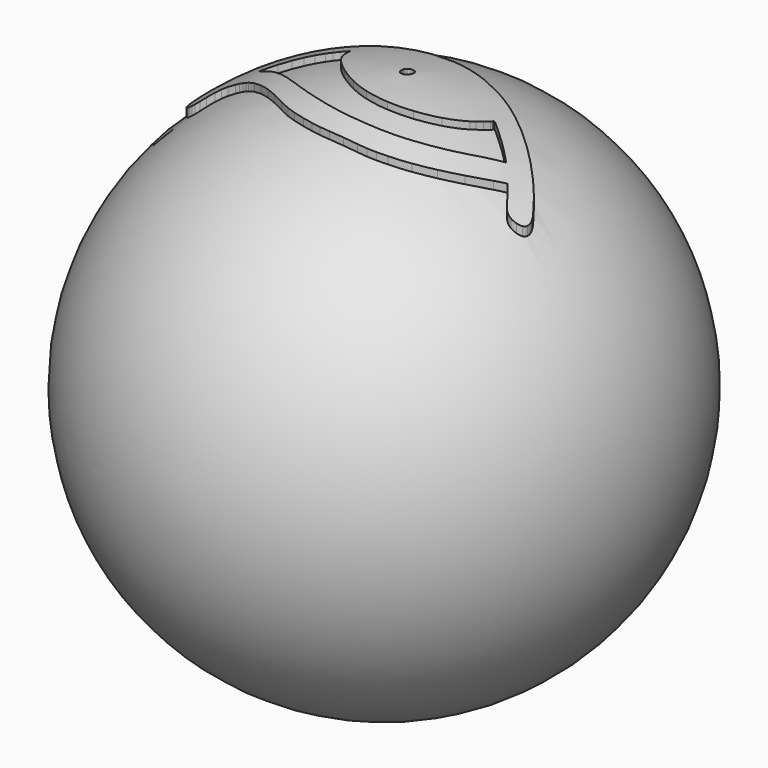
from build123d import *

# Parameters (mm, degrees)
F2_SCALE  = 33.3
F4_DEPTH  = 350
F5_SCALE  = 0.03
F8_SCALE  = 1.4
F9_R      = 2
F10_DEPTH = 25


# Not quite as in the source:
# - ends of sketch curves that miss each other by under 0.0002 mm in the source are joined


with BuildPart() as f1:
    # F0 (on Top) → F1 (revolve)
    with BuildSketch(Plane.XY):
        with BuildLine():
            ThreePointArc((0, 10), (-10, 0), (0, -10))
            Line((0, -10), (0, 10))
        make_face()
    revolve(axis=Axis((0, 0, 0), (0, 1, 0)))


with BuildPart() as f1_1:
    # F2: moved
    add(f1.part.scale(F2_SCALE))

    # F3 (on Top) → F4 (join)
    with BuildSketch(Plane.XY):
        with BuildLine():
            ThreePointArc((10.0534840034, 96.9614781182), (-2.8301346595, 96.9747207616), (-15.6947390095, 96.2748921162))
            ThreePointArc((-15.6947390095, 96.2748921162), (-24.8751298312, 95.2803343458), (-33.991766952, 93.8121217445))
            ThreePointArc((-33.991766952, 93.8121217445), (-43.5504868945, 91.8004399256), (-53.0120990138, 89.3727070494))
            ThreePointArc((-53.0120990138, 89.3727070494), (-62.3941886789, 86.5234517907), (-71.6431770265, 83.2679830704))
            ThreePointArc((-71.6431770265, 83.2679830704), (-80.3024909146, 79.7548321438), (-88.7739972032, 75.8102754091))
            ThreePointArc((-88.7739972032, 75.8102754091), (-102.8123104581, 68.2085488829), (-116.2787087414, 59.6343666239))
            ThreePointArc((-116.2787087414, 59.6343666239), (-129.8649070153, 49.6780948633), (-142.827490195, 38.9224652211))
            ThreePointArc((-142.827490195, 38.9224652211), (-156.8673095819, 25.8818104455), (-170.2157531103, 12.1342921017))
            ThreePointArc((-170.2157531103, 12.1342921017), (-185.5506121287, -5.0061794181), (-200.3640161811, -22.5992668521))
            ThreePointArc((-200.3640161811, -22.5992668521), (-204.2556653518, -27.3979139103), (-208.1144591023, -32.2230209187))
            ThreePointArc((-208.1144591023, -32.2230209187), (-209.6806871871, -34.3340096505), (-211.1049830246, -36.5432459852))
            ThreePointArc((-211.1049830246, -36.5432459852), (-211.8903487056, -38.1080067712), (-212.4343023025, -39.7721551716))
            ThreePointArc((-212.4343023025, -39.7721551716), (-212.7727330789, -41.6217988462), (-212.886093, -43.498729))
            ThreePointArc((-212.886093, -43.498729), (-212.7053479315, -45.3625594436), (-212.1698450767, -47.1569310312))
            ThreePointArc((-212.1698450767, -47.1569310312), (-211.2496275997, -49.0288969817), (-210.0765223808, -50.7536813001))
            ThreePointArc((-210.0765223808, -50.7536813001), (-208.6303513581, -52.3522530467), (-206.981032979, -53.7402699713))
            ThreePointArc((-206.981032979, -53.7402699713), (-205.2320729108, -54.8208646921), (-203.3361079867, -55.6157629597))
            ThreePointArc((-203.3361079867, -55.6157629597), (-201.3422328116, -56.0863212361), (-199.2969970047, -56.2045318412))
            ThreePointArc((-199.2969970047, -56.2045318412), (-197.4275801661, -55.9408822607), (-195.6618639687, -55.2726930612))
            ThreePointArc((-195.6618639687, -55.2726930612), (-193.6718494664, -54.0492698967), (-191.8979606388, -52.52932236))
            ThreePointArc((-191.8979606388, -52.52932236), (-189.5399689495, -50.0368818855), (-187.3149011588, -47.4250898717))
            ThreePointArc((-187.3149011588, -47.4250898717), (-184.5776350656, -44.2864403575), (-181.612206547, -41.3624054954))
            ThreePointArc((-181.612206547, -41.3624054954), (-179.0131248493, -39.3175211967), (-176.1404878573, -37.6790052998))
            ThreePointArc((-176.1404878573, -37.6790052998), (-172.9686200832, -36.4355960849), (-169.65328502, -35.6511438773))
            ThreePointArc((-169.65328502, -35.6511438773), (-165.1982751687, -35.067458336), (-160.7153950073, -34.7648247958))
            ThreePointArc((-160.7153950073, -34.7648247958), (-158.1528140465, -34.7037638823), (-155.5895059941, -34.7049725349))
            ThreePointArc((-155.5895059941, -34.7049725349), (-153.4579068829, -34.7765835211), (-151.3311820401, -34.9374694148))
            ThreePointArc((-151.3311820401, -34.9374694148), (-149.2878923738, -35.180741935), (-147.2573030885, -35.5137904739))
            ThreePointArc((-147.2573030885, -35.5137904739), (-144.9787497299, -35.975458744), (-142.7153951261, -36.5066545025))
            ThreePointArc((-142.7153951261, -36.5066545025), (-137.7060507754, -37.9788293633), (-132.8304160593, -39.8467201381))
            ThreePointArc((-132.8304160593, -39.8467201381), (-126.177935546, -42.8259254875), (-119.6189671008, -46.0057202002))
            ThreePointArc((-119.6189671008, -46.0057202002), (-111.9353070881, -50.0083471014), (-104.3637867666, -54.2192535934))
            ThreePointArc((-104.3637867666, -54.2192535934), (-96.07539311, -59.0890561452), (-87.8860931987, -64.1237173161))
            ThreePointArc((-87.8860931987, -64.1237173161), (-78.6401870334, -69.8346933419), (-69.3050959968, -75.3986939946))
            ThreePointArc((-69.3050959968, -75.3986939946), (-62.777455601, -79.0174912251), (-56.0877589877, -82.3271349735))
            ThreePointArc((-56.0877589877, -82.3271349735), (-50.0824455847, -84.916376715), (-43.9372820283, -87.1535460853))
            ThreePointArc((-43.9372820283, -87.1535460853), (-36.7011886725, -89.4037622878), (-29.3860929668, -91.3821188674))
            ThreePointArc((-29.3860929668, -91.3821188674), (-22.7529677477, -92.9483569917), (-16.0797740003, -94.3339750015))
            ThreePointArc((-16.0797740003, -94.3339750015), (-10.39619629, -95.3028132915), (-4.6750499334, -96.0170873481))
            ThreePointArc((-4.6750499334, -96.0170873481), (1.6922174435, -96.5465813773), (8.0749579989, -96.8348190408))
            ThreePointArc((8.0749579989, -96.8348190408), (17.0936610047, -97.008448933), (26.113906999, -97.0565464094))
            ThreePointArc((26.113906999, -97.0565464094), (34.8126763388, -96.981346949), (43.5095330001, -96.7840470048))
            ThreePointArc((43.5095330001, -96.7840470048), (49.3823217448, -96.482178626), (55.2365339914, -95.9263269263))
            ThreePointArc((55.2365339914, -95.9263269263), (60.4241703797, -95.1815075627), (65.5655091121, -94.1651594979))
            ThreePointArc((65.5655091121, -94.1651594979), (71.7311409903, -92.6799724172), (77.8496770529, -91.011346183))
            ThreePointArc((77.8496770529, -91.011346183), (89.6484081947, -87.0836085971), (101.0937568624, -82.2213897092))
            ThreePointArc((101.0937568624, -82.2213897092), (112.524177247, -76.2978835685), (123.495907726, -69.5626355879))
            ThreePointArc((123.495907726, -69.5626355879), (134.4761853274, -61.7039148815), (144.8899505352, -53.1085974748))
            ThreePointArc((144.8899505352, -53.1085974748), (155.2993648009, -43.341260859), (165.1221510548, -32.9841550491))
            Line((165.1221510548, -32.9841550491), (174.59639, -22.392832))
            Line((174.59639, -22.392832), (177.927907, -26.246049))
            ThreePointArc((177.927907, -26.246049), (178.757510393, -27.2335755521), (179.5587290452, -28.2442679652))
            ThreePointArc((179.5587290452, -28.2442679652), (180.6874722444, -29.7254244326), (181.8016047585, -31.2176021785))
            ThreePointArc((181.8016047585, -31.2176021785), (183.0140394599, -32.8750469761), (184.2102467845, -34.5442411529))
            ThreePointArc((184.2102467845, -34.5442411529), (185.3325359305, -36.1456252327), (186.436664797, -37.7595841372))
            ThreePointArc((186.436664797, -37.7595841372), (188.8872919195, -41.1685808828), (191.5310503706, -44.4300795411))
            ThreePointArc((191.5310503706, -44.4300795411), (193.4908629635, -46.2905329442), (195.7849111403, -47.7186417136))
            ThreePointArc((195.7849111403, -47.7186417136), (197.9411085364, -48.4270922813), (200.2087749936, -48.5207849344))
            ThreePointArc((200.2087749936, -48.5207849344), (202.9674262395, -48.0428871064), (205.624129238, -47.1594435696))
            ThreePointArc((205.624129238, -47.1594435696), (208.3096237637, -45.6184315237), (210.5296332459, -43.4601551966))
            ThreePointArc((210.5296332459, -43.4601551966), (212.0446506291, -40.8973126926), (212.789883761, -38.014940973))
            ThreePointArc((212.789883761, -38.014940973), (212.7878168698, -34.5816998907), (212.0153318509, -31.2364920528))
            ThreePointArc((212.0153318509, -31.2364920528), (210.3771533117, -27.4070249468), (208.2627591594, -23.8184618918))
            ThreePointArc((208.2627591594, -23.8184618918), (196.5741889553, -8.0121673939), (183.6542946789, 6.8046456965))
            ThreePointArc((183.6542946789, 6.8046456965), (168.5057313524, 21.8538564549), (152.4429349281, 35.9231239125))
            ThreePointArc((152.4429349281, 35.9231239125), (135.4811978341, 48.9959528787), (117.7344819259, 60.9815048825))
            ThreePointArc((117.7344819259, 60.9815048825), (100.5483373809, 70.8981711943), (82.6359109068, 79.4333227827))
            ThreePointArc((82.6359109068, 79.4333227827), (70.0438254204, 84.474375404), (57.2196661308, 88.8918144124))
            ThreePointArc((57.2196661308, 88.8918144124), (45.5557201871, 92.1552038245), (33.6950569547, 94.6091827356))
            ThreePointArc((33.6950569547, 94.6091827356), (21.9157214443, 96.20193026), (10.0534840034, 96.9614781182))
        make_face()
        with BuildLine():
            ThreePointArc((-82.927290334, 48.3948199687), (-82.8826026832, 47.7734545619), (-82.8650012937, 47.1507329981))
            ThreePointArc((-82.8650012937, 47.1507329981), (-82.8223320769, 46.3055581613), (-82.7056262352, 45.4673929566))
            ThreePointArc((-82.7056262352, 45.4673929566), (-82.4536217423, 44.1929730018), (-82.1687810713, 42.925487983))
            ThreePointArc((-82.1687810713, 42.925487983), (-81.8096255262, 41.5001455931), (-81.4139185569, 40.08451513))
            ThreePointArc((-81.4139185569, 40.08451513), (-80.9877809683, 38.7016352496), (-80.524508707, 37.3307491034))
            ThreePointArc((-80.524508707, 37.3307491034), (-75.9793443062, 27.4848022568), (-69.6898092464, 18.6506107875))
            ThreePointArc((-69.6898092464, 18.6506107875), (-60.1843703175, 8.5972984948), (-49.8032193252, -0.5489664049))
            ThreePointArc((-49.8032193252, -0.5489664049), (-38.0813797686, -9.135101843), (-25.6433221245, -16.6462912285))
            ThreePointArc((-25.6433221245, -16.6462912285), (-13.9136781439, -22.1115037248), (-1.5919049769, -26.0646039086))
            ThreePointArc((-1.5919049769, -26.0646039086), (12.8223370252, -28.6094128934), (27.4533770014, -29.0326090321))
            ThreePointArc((27.4533770014, -29.0326090321), (42.1444954977, -27.3399258677), (56.4503389882, -23.5933299652))
            ThreePointArc((56.4503389882, -23.5933299652), (69.7851613505, -17.9667617613), (82.1681429973, -10.4742639962))
            ThreePointArc((82.1681429973, -10.4742639962), (92.7301684437, -1.5801003949), (101.670577089, 8.9428089363))
            ThreePointArc((101.670577089, 8.9428089363), (103.4699853461, 11.5910326673), (105.1395603107, 14.3229693988))
            ThreePointArc((105.1395603107, 14.3229693988), (107.1272029408, 17.8564119714), (109.0292600758, 21.4366519609))
            ThreePointArc((109.0292600758, 21.4366519609), (110.7947025287, 24.9242841932), (112.5060959137, 28.4387540412))
            ThreePointArc((112.5060959137, 28.4387540412), (112.9600537039, 29.7466541413), (113.113907, 31.122521))
            ThreePointArc((113.113907, 31.122521), (113.1284819934, 31.3686596395), (113.1720039652, 31.6113580084))
            ThreePointArc((113.1720039652, 31.6113580084), (113.2415255349, 31.8250069213), (113.343400909, 32.0252580556))
            ThreePointArc((113.343400909, 32.0252580556), (113.4568935563, 32.1761316229), (113.5971697595, 32.3024883251))
            ThreePointArc((113.5971697595, 32.3024883251), (113.7382778168, 32.3755381569), (113.895163, 32.400733))
            ThreePointArc((113.895163, 32.400733), (115.0187308209, 32.2140806192), (116.0215990284, 31.6741740367))
            ThreePointArc((116.0215990284, 31.6741740367), (122.3839566736, 26.7345530401), (128.7296019892, 21.7734809863))
            ThreePointArc((128.7296019892, 21.7734809863), (134.7052209765, 17.0276272722), (140.6238469382, 12.210883925))
            ThreePointArc((140.6238469382, 12.210883925), (144.6717950827, 8.7595987557), (148.6006183995, 5.1732913641))
            Line((148.6006183995, 5.1732913641), (157.58733, -3.313212))
            Line((157.58733, -3.313212), (142.600619, -18.24085))
            ThreePointArc((142.600619, -18.24085), (136.7807196618, -23.8941575955), (130.8208438643, -29.3996998494))
            ThreePointArc((130.8208438643, -29.3996998494), (125.6669555944, -33.8487564835), (120.3298188274, -38.0762427724))
            ThreePointArc((120.3298188274, -38.0762427724), (115.1679134871, -41.806229524), (109.839608073, -45.2943851173))
            ThreePointArc((109.839608073, -45.2943851173), (104.0414742659, -48.7480108155), (98.113907386, -51.974438743))
            ThreePointArc((98.113907386, -51.974438743), (90.086932018, -55.8855797642), (81.8696532409, -59.3792436096))
            ThreePointArc((81.8696532409, -59.3792436096), (73.9747685825, -62.2196229737), (65.9192639068, -64.5660676387))
            ThreePointArc((65.9192639068, -64.5660676387), (57.6485454123, -66.4322374111), (49.2792660567, -67.7896384328))
            ThreePointArc((49.2792660567, -67.7896384328), (40.1375655488, -68.7644368063), (30.9596300226, -69.2996186587))
            ThreePointArc((30.9596300226, -69.2996186587), (21.9460062425, -69.4151836268), (12.9357099866, -69.14438826))
            ThreePointArc((12.9357099866, -69.14438826), (4.356760116, -68.4900668727), (-4.1795320796, -67.4138545265))
            ThreePointArc((-4.1795320796, -67.4138545265), (-12.7642691218, -65.9019463311), (-21.2655348698, -63.975276484))
            ThreePointArc((-21.2655348698, -63.975276484), (-30.2875406451, -61.509472013), (-39.2056621797, -58.6909815319))
            ThreePointArc((-39.2056621797, -58.6909815319), (-46.1452229248, -56.2463133395), (-53.0191921884, -53.622870475))
            ThreePointArc((-53.0191921884, -53.622870475), (-59.2414418849, -51.0334594382), (-65.3730498874, -48.2361707638))
            ThreePointArc((-65.3730498874, -48.2361707638), (-72.4013590577, -44.7698153352), (-79.3345330974, -41.116892179))
            ThreePointArc((-79.3345330974, -41.116892179), (-89.0822827657, -35.7521524082), (-98.7776571539, -30.2933272703))
            ThreePointArc((-98.7776571539, -30.2933272703), (-106.3799678778, -26.033668345), (-114.0404019282, -21.8794448653))
            ThreePointArc((-114.0404019282, -21.8794448653), (-119.864757432, -18.891230375), (-125.7815339819, -16.0904629602))
            ThreePointArc((-125.7815339819, -16.0904629602), (-130.7256731817, -13.9673363184), (-135.7528159623, -12.0489998948))
            ThreePointArc((-135.7528159623, -12.0489998948), (-140.5059156849, -10.4817808164), (-145.3327459719, -9.1589648862))
            Line((-145.3327459719, -9.1589648862), (-154.279399, -6.95077))
            Line((-154.279399, -6.95077), (-140.332746, 6.994467))
            ThreePointArc((-140.332746, 6.994467), (-135.3781172255, 11.8749363674), (-130.3509390015, 16.6806420016))
            ThreePointArc((-130.3509390015, 16.6806420016), (-125.9578414585, 20.7208736929), (-121.4705605604, 24.6562374867))
            ThreePointArc((-121.4705605604, 24.6562374867), (-117.3140423165, 28.1212004675), (-113.0671904207, 31.4748345476))
            ThreePointArc((-113.0671904207, 31.4748345476), (-108.8544622177, 34.6159831895), (-104.5526307339, 37.6339526088))
            ThreePointArc((-104.5526307339, 37.6339526088), (-101.4481052436, 39.7141793365), (-98.3149537113, 41.7510355491))
            ThreePointArc((-98.3149537113, 41.7510355491), (-94.9120280604, 43.9031758716), (-91.4853724929, 46.0173288089))
            ThreePointArc((-91.4853724929, 46.0173288089), (-88.177257622, 48.0248032611), (-84.8618779652, 50.0202569419))
            ThreePointArc((-84.8618779652, 50.0202569419), (-84.2720055563, 50.2782386341), (-83.6360930038, 50.3788331317))
            ThreePointArc((-83.6360930038, 50.3788331317), (-83.4605806472, 50.3298015447), (-83.3438589327, 50.1898560279))
            ThreePointArc((-83.3438589327, 50.1898560279), (-83.2071078188, 49.8195815839), (-83.1002097877, 49.4396120507))
            ThreePointArc((-83.1002097877, 49.4396120507), (-82.9953397503, 48.9202630179), (-82.927290334, 48.3948199687))
        make_face(mode=Mode.SUBTRACT)
        with BuildLine():
            ThreePointArc((5.6446279231, 39.9987247815), (6.8074154783, 39.4980422554), (7.891400803, 38.8440287187))
            ThreePointArc((7.891400803, 38.8440287187), (8.4497152592, 38.3972254722), (8.9465351952, 37.8829121658))
            ThreePointArc((8.9465351952, 37.8829121658), (9.3324485382, 37.3462719051), (9.6270404866, 36.754556195))
            ThreePointArc((9.6270404866, 36.754556195), (9.8608059068, 36.0370138043), (9.9977493569, 35.2948819249))
            ThreePointArc((9.9977493569, 35.2948819249), (10.0848428304, 34.298416225), (10.113907, 33.298574))
            ThreePointArc((10.113907, 33.298574), (9.6686317016, 30.3700248444), (8.373047846, 27.7061681062))
            ThreePointArc((8.373047846, 27.7061681062), (6.4189182148, 25.7723202075), (3.8932430958, 24.6863385697))
            ThreePointArc((3.8932430958, 24.6863385697), (1.4915347311, 24.7266396179), (-0.6296868515, 25.8536911679))
            ThreePointArc((-0.6296868515, 25.8536911679), (-2.2074961218, 27.9068574867), (-2.9043163097, 30.4007330561))
            ThreePointArc((-2.9043163097, 30.4007330561), (-2.9960622325, 31.8974630018), (-3.0282842145, 33.3966559997))
            ThreePointArc((-3.0282842145, 33.3966559997), (-2.9636646702, 34.3686478157), (-2.7678425193, 35.322900144))
            ThreePointArc((-2.7678425193, 35.322900144), (-2.4733140871, 36.1087811962), (-2.045497151, 36.8308121085))
            ThreePointArc((-2.045497151, 36.8308121085), (-1.4093806412, 37.6296348848), (-0.6975319731, 38.3617779711))
            ThreePointArc((-0.6975319731, 38.3617779711), (0.2601182339, 39.1314654839), (1.3195740848, 39.753611828))
            ThreePointArc((1.3195740848, 39.753611828), (2.3530427174, 40.1396585124), (3.442768025, 40.3116705546))
            ThreePointArc((3.442768025, 40.3116705546), (4.5591822042, 40.2641434744), (5.6446279231, 39.9987247815))
        make_face(mode=Mode.SUBTRACT)
    extrude(amount=F4_DEPTH)


with BuildPart() as f1_2:
    # F5: moved
    add(f1_1.part.scale(F5_SCALE))

    # F6 (on Top) → F7 (revolve, cut)
    with BuildSketch(Plane.XY):
        with BuildLine():
            Line((0, 10.25), (0, 15))
            ThreePointArc((0, 15), (-15, 0), (0, -15))
            Line((0, -15), (0, -10.25))
            ThreePointArc((0, -10.25), (-10.25, 0), (0, 10.25))
        make_face()
        with BuildLine():
            Line((0, -7), (0, 7))
            ThreePointArc((0, 7), (-7, 0), (0, -7))
        make_face()
    revolve(axis=Axis((0, 0, 0), (0, -1, 0)), mode=Mode.SUBTRACT)


with BuildPart() as f1_3:
    # F8: moved
    add(f1_2.part.scale(F8_SCALE))

    # F9 (on Front) → F10 (cut)
    with BuildSketch(Plane.XZ):
        with Locations((0, -5.1200183504)):
            Circle(F9_R)
    extrude(amount=-F10_DEPTH, mode=Mode.SUBTRACT)


solid = f1_3.part
